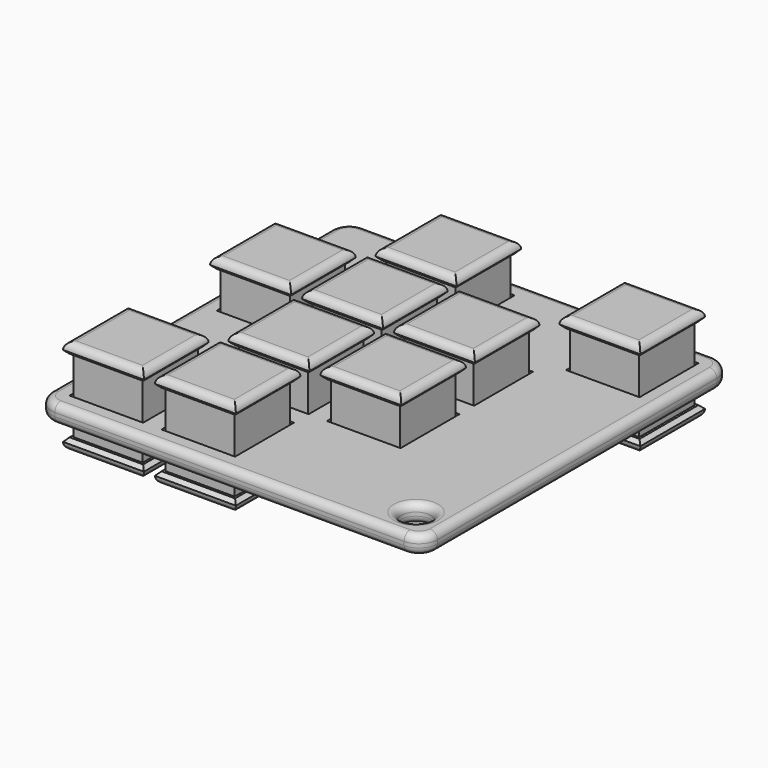
from build123d import *

# Parameters (mm, degrees)
F0_W     = 9.3999998644
F0_H     = 9.3999998644
F1_DEPTH = 5
F0_W_2   = 10
F0_H_2   = 10
F0_R     = 2
F2_DEPTH = 2.5
F3_W     = 11
F3_H     = 11
F4_DEPTH = 1.5
F3_W_2   = 9.3999998644
F3_H_2   = 9.3999998644
F6_SIZE  = 0.5
F7_R     = 0.99999
F7_2_R   = 0.99999


# Not quite as in the source:
# - a fillet or chamfer is up to 0.001 mm smaller than in the source, because OpenCascade refuses the exact size


with BuildPart() as f1:
    # F0 (on Top) → F1 (new body, symmetric)
    with BuildSketch(Plane.XY):
        Rectangle(F0_W, F0_H)
    extrude(amount=F1_DEPTH, both=True)

    # F3 (on face) → F4, piece 9 (join)
    with BuildSketch(Plane.XY.offset(5)):
        Rectangle(F3_W, F3_H)
        Rectangle(F3_W_2, F3_H_2, mode=Mode.SUBTRACT)
        Rectangle(F3_W_2, F3_H_2)
    extrude(amount=F4_DEPTH)



with BuildPart() as f1b:
    # F0 (on Top) → F1, piece 2 (new body, symmetric)
    with BuildSketch(Plane.XY):
        with Locations((12.5, 0)):
            Rectangle(F0_W, F0_H)
    extrude(amount=F1_DEPTH, both=True)

    # F3 (on face) → F4, piece 2 (join)
    with BuildSketch(Plane.XY.offset(5)):
        with Locations((12.5, 0)):
            Rectangle(F3_W, F3_H)
    extrude(amount=F4_DEPTH)


with BuildPart() as f1c:
    # F0 (on Top) → F1, piece 3 (new body, symmetric)
    with BuildSketch(Plane.XY):
        with Locations((12.5, 12.5)):
            Rectangle(F0_W, F0_H)
    extrude(amount=F1_DEPTH, both=True)

    # F3 (on face) → F4, piece 3 (join)
    with BuildSketch(Plane.XY.offset(5)):
        with Locations((12.5, 12.5)):
            Rectangle(F3_W, F3_H)
    extrude(amount=F4_DEPTH)


with BuildPart() as f1d:
    # F0 (on Top) → F1, piece 4 (new body, symmetric)
    with BuildSketch(Plane.XY):
        with Locations((25, 12.5)):
            Rectangle(F0_W, F0_H)
    extrude(amount=F1_DEPTH, both=True)

    # F3 (on face) → F4, piece 8 (join)
    with BuildSketch(Plane.XY.offset(5)):
        with Locations((25, 12.5)):
            Rectangle(F3_W, F3_H)
    extrude(amount=F4_DEPTH)


with BuildPart() as f1e:
    # F0 (on Top) → F1, piece 5 (new body, symmetric)
    with BuildSketch(Plane.XY):
        with Locations((25, 25)):
            Rectangle(F0_W, F0_H)
    extrude(amount=F1_DEPTH, both=True)

    # F3 (on face) → F4, piece 7 (join)
    with BuildSketch(Plane.XY.offset(5)):
        with Locations((25, 25)):
            Rectangle(F3_W, F3_H)
    extrude(amount=F4_DEPTH)


with BuildPart() as f1f:
    # F0 (on Top) → F1, piece 6 (new body, symmetric)
    with BuildSketch(Plane.XY):
        with Locations((12.5, 25)):
            Rectangle(F0_W, F0_H)
    extrude(amount=F1_DEPTH, both=True)

    # F3 (on face) → F4, piece 4 (join)
    with BuildSketch(Plane.XY.offset(5)):
        with Locations((12.5, 25)):
            Rectangle(F3_W, F3_H)
    extrude(amount=F4_DEPTH)


with BuildPart() as f1g:
    # F0 (on Top) → F1, piece 7 (new body, symmetric)
    with BuildSketch(Plane.XY):
        with Locations((0, 25)):
            Rectangle(F0_W, F0_H)
    extrude(amount=F1_DEPTH, both=True)

    # F3 (on face) → F4 (join)
    with BuildSketch(Plane.XY.offset(5)):
        with Locations((0, 25)):
            Rectangle(F3_W, F3_H)
    extrude(amount=F4_DEPTH)


with BuildPart() as f1h:
    # F0 (on Top) → F1, piece 8 (new body, symmetric)
    with BuildSketch(Plane.XY):
        with Locations((37.5, 37.5)):
            Rectangle(F0_W, F0_H)
    extrude(amount=F1_DEPTH, both=True)

    # F3 (on face) → F4, piece 6 (join)
    with BuildSketch(Plane.XY.offset(5)):
        with Locations((37.5, 37.5)):
            Rectangle(F3_W, F3_H)
    extrude(amount=F4_DEPTH)


with BuildPart() as f1i:
    # F0 (on Top) → F1, piece 9 (new body, symmetric)
    with BuildSketch(Plane.XY):
        with Locations((12.5, 37.5)):
            Rectangle(F0_W, F0_H)
    extrude(amount=F1_DEPTH, both=True)

    # F3 (on face) → F4, piece 5 (join)
    with BuildSketch(Plane.XY.offset(5)):
        with Locations((12.5, 37.5)):
            Rectangle(F3_W, F3_H)
    extrude(amount=F4_DEPTH)


with BuildPart() as f2:
    # F0 (on Top) → F2 (new body)
    with BuildSketch(Plane.XY):
        with BuildLine():
            ThreePointArc((-7.5, -5), (-6.767766953, -6.767766953), (-5, -7.5))
            Line((-5, -7.5), (42.5, -7.5))
            ThreePointArc((42.5, -7.5), (44.267766953, -6.767766953), (45, -5))
            Line((45, -5), (45, 42.5))
            ThreePointArc((45, 42.5), (44.267766953, 44.267766953), (42.5, 45))
            Line((42.5, 45), (-5, 45))
            ThreePointArc((-5, 45), (-6.767766953, 44.267766953), (-7.5, 42.5))
            Line((-7.5, 42.5), (-7.5, -5))
        make_face()
        Rectangle(F0_W_2, F0_H_2, mode=Mode.SUBTRACT)
        with Locations((12.5, 0)):
            Rectangle(F0_W_2, F0_H_2, mode=Mode.SUBTRACT)
        with Locations((12.5, 12.5)):
            Rectangle(F0_W_2, F0_H_2, mode=Mode.SUBTRACT)
        with Locations((40.5, -3)):
            Circle(F0_R, mode=Mode.SUBTRACT)
        with Locations((25, 12.5)):
            Rectangle(F0_W_2, F0_H_2, mode=Mode.SUBTRACT)
        with Locations((0, 25)):
            Rectangle(F0_W_2, F0_H_2, mode=Mode.SUBTRACT)
        with Locations((12.5, 25)):
            Rectangle(F0_W_2, F0_H_2, mode=Mode.SUBTRACT)
        with Locations((12.5, 37.5)):
            Rectangle(F0_W_2, F0_H_2, mode=Mode.SUBTRACT)
        with Locations((25, 25)):
            Rectangle(F0_W_2, F0_H_2, mode=Mode.SUBTRACT)
        with Locations((37.5, 37.5)):
            Rectangle(F0_W_2, F0_H_2, mode=Mode.SUBTRACT)
    extrude(amount=-F2_DEPTH)

    # F7 (radius 1 in the source; OpenCascade refuses exactly that, so slightly less here)
    f7_edges = [f2.edges().sort_by_distance(p)[0] for p in [
        (18.75, -7.5, -2.5),
        (44.267767, -6.767767, -2.5),
        (45, 18.75, -2.5),
        (-6.767767, -6.767767, -2.5),
        (-6.767767, 44.267767, -2.5),
        (44.267767, 44.267767, -2.5),
        (18.75, 45, -2.5),
        (-7.5, 18.75, 0),
        (38.5, -3, -2.5),
        (38.5, -3, 0),
    ]]
    fillet(f7_edges, radius=F7_R)


with BuildPart() as f1_1:
    add(f1.part)

    add(f1b.part)  # F5 merges F1b

    add(f1c.part)  # F5 merges F1c

    add(f1d.part)  # F5 merges F1d

    add(f1e.part)  # F5 merges F1e

    add(f1f.part)  # F5 merges F1f

    add(f1g.part)  # F5 merges F1g

    add(f1h.part)  # F5 merges F1h

    add(f1i.part)  # F5 merges F1i
    # F5: F1g, F1b, F1c, F1f, F1i, F1h, F1e, F1d, F1 across plane
    add(f1g.part.mirror(Plane.XY))
    add(f1b.part.mirror(Plane.XY))
    add(f1c.part.mirror(Plane.XY))
    add(f1f.part.mirror(Plane.XY))
    add(f1i.part.mirror(Plane.XY))
    add(f1h.part.mirror(Plane.XY))
    add(f1e.part.mirror(Plane.XY))
    add(f1d.part.mirror(Plane.XY))
    add(f1.part.mirror(Plane.XY))

    # F6
    f6_edges = [f1_1.edges().sort_by_distance(p)[0] for p in [
        (37.5, 43, 5),
        (12.5, 43, 5),
        (32, 37.5, 5),
        (7, 37.5, 5),
        (12.5, 30.5, 5),
        (7, 25, 5),
        (0, 30.5, 5),
        (-5.5, 25, 5),
        (7, 12.5, 5),
        (12.5, 5.5, 5),
        (0, 5.5, 5),
        (-5.5, 0, 5),
        (7, 0, 5),
        (12.5, 18, 5),
        (25, 18, 5),
        (25, 30.5, 5),
        (19.5, 25, 5),
        (19.5, 12.5, 5),
        (37.5, 43, -5),
        (32, 37.5, -5),
        (12.5, 43, -5),
        (7, 37.5, -5),
        (0, 30.5, -5),
        (-5.5, 25, -5),
        (0, 5.5, -5),
        (-5.5, 0, -5),
        (0, -5.5, -5),
        (7, 0, -5),
        (12.5, -5.5, -5),
        (12.5, -5.5, 5),
        (0, 19.5, 5),
        (25, 7, 5),
        (0, -5.5, 5),
        (12.5, 32, 5),
        (12.5, 19.5, 5),
        (25, 19.5, 5),
        (18, 0, -5),
        (18, 12.5, -5),
        (12.5, 7, -5),
        (25, 7, -5),
        (30.5, 12.5, -5),
        (18, 0, 5),
        (30.5, 12.5, 5),
        (30.5, 25, 5),
        (12.5, 7, 5),
        (18, 12.5, 5),
        (18, 25, 5),
        (5.5, 0, 5),
        (5.5, 25, 5),
        (18, 37.5, 5),
        (43, 37.5, 5),
        (37.5, 32, 5),
        (18, 37.5, -5),
        (12.5, 32, -5),
        (37.5, 32, -5),
        (43, 37.5, -5),
        (30.5, 25, -5),
        (25, 30.5, -5),
        (19.5, 25, -5),
        (25, 19.5, -5),
        (25, 18, -5),
        (12.5, 5.5, -5),
        (12.5, 18, -5),
        (18, 25, -5),
        (12.5, 30.5, -5),
        (19.5, 12.5, -5),
        (7, 25, -5),
        (7, 12.5, -5),
        (12.5, 19.5, -5),
        (5.5, 0, -5),
        (0, 19.5, -5),
        (5.5, 25, -5),
    ]]
    chamfer(f6_edges, length=F6_SIZE)

    # F7#2 (radius 1 in the source; OpenCascade refuses exactly that, so slightly less here)
    f7_2_edges = [f1_1.edges().sort_by_distance(p)[0] for p in [
        (18, 37.5, -6.5),
        (12.5, 43, -6.5),
        (7, 37.5, -6.5),
        (12.5, 32, -6.5),
        (18, 25, -6.5),
        (12.5, 30.5, -6.5),
        (7, 25, -6.5),
        (12.5, 19.5, -6.5),
        (30.5, 25, -6.5),
        (25, 30.5, -6.5),
        (19.5, 25, -6.5),
        (25, 19.5, -6.5),
        (43, 37.5, -6.5),
        (37.5, 43, -6.5),
        (32, 37.5, -6.5),
        (37.5, 32, -6.5),
        (30.5, 12.5, -6.5),
        (25, 18, -6.5),
        (19.5, 12.5, -6.5),
        (25, 7, -6.5),
        (18, 12.5, -6.5),
        (12.5, 18, -6.5),
        (7, 12.5, -6.5),
        (12.5, 7, -6.5),
        (18, 0, -6.5),
        (12.5, 5.5, -6.5),
        (7, 0, -6.5),
        (12.5, -5.5, -6.5),
        (5.5, 0, -6.5),
        (0, 5.5, -6.5),
        (-5.5, 0, -6.5),
        (0, -5.5, -6.5),
        (5.5, 25, -6.5),
        (0, 30.5, -6.5),
        (-5.5, 25, -6.5),
        (0, 19.5, -6.5),
        (18, 0, 6.5),
        (12.5, 5.5, 6.5),
        (7, 0, 6.5),
        (12.5, -5.5, 6.5),
        (5.5, 0, 6.5),
        (0, 5.5, 6.5),
        (-5.5, 0, 6.5),
        (0, -5.5, 6.5),
        (18, 12.5, 6.5),
        (12.5, 18, 6.5),
        (7, 12.5, 6.5),
        (12.5, 7, 6.5),
        (30.5, 12.5, 6.5),
        (25, 18, 6.5),
        (19.5, 12.5, 6.5),
        (25, 7, 6.5),
        (30.5, 25, 6.5),
        (25, 30.5, 6.5),
        (19.5, 25, 6.5),
        (25, 19.5, 6.5),
        (43, 37.5, 6.5),
        (37.5, 43, 6.5),
        (32, 37.5, 6.5),
        (37.5, 32, 6.5),
        (18, 37.5, 6.5),
        (12.5, 43, 6.5),
        (7, 37.5, 6.5),
        (12.5, 32, 6.5),
        (5.5, 25, 6.5),
        (0, 30.5, 6.5),
        (-5.5, 25, 6.5),
        (0, 19.5, 6.5),
        (18, 25, 6.5),
        (12.5, 30.5, 6.5),
        (7, 25, 6.5),
        (12.5, 19.5, 6.5),
    ]]
    fillet(f7_2_edges, radius=F7_2_R)


solid = Compound([f2.part, f1_1.part])
